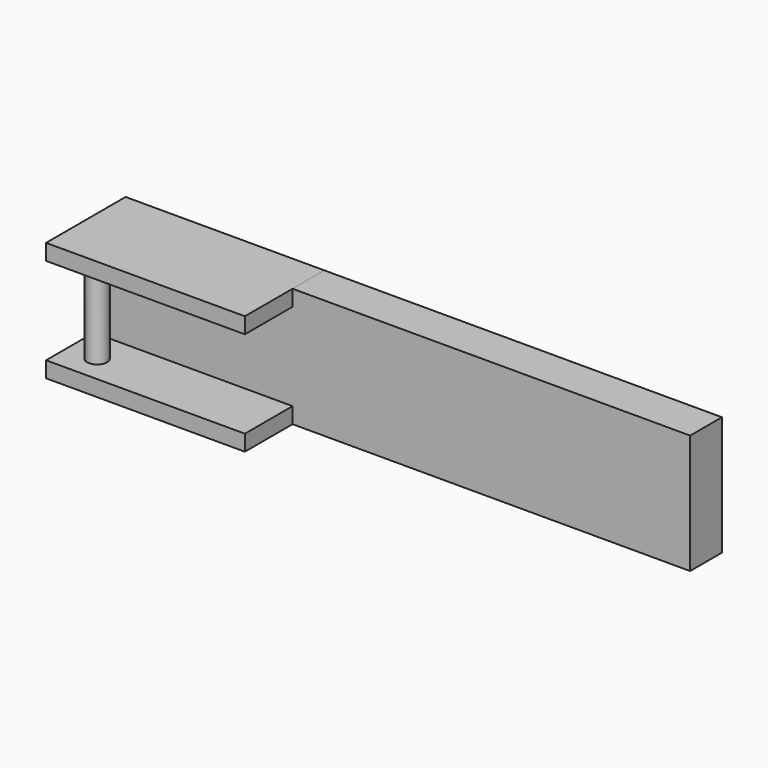
from build123d import *

# Parameters (mm, degrees)
F0_W     = 63.5
F0_H     = 5.08
F1_DEPTH = 31.75
F0_H_2   = 27.94
F2_DEPTH = 12.7
F3_R     = 3.175
F4_DEPTH = 28.702


with BuildPart() as f1:
    # F0 (on Front) → F1 (new body)
    with BuildSketch(Plane.XZ):
        with Locations((-63.5, 16.51)):
            Rectangle(F0_W, F0_H)
    extrude(amount=F1_DEPTH)

    # F3 (on face) → F4 (join)
    with BuildSketch(Plane(origin=(0, 0, 13.97), x_dir=(1, 0, 0), z_dir=(0, 0, -1))):
        with Locations((-85.8540832996, 23.1188889593)):
            Circle(F3_R)
    extrude(amount=F4_DEPTH)


with BuildPart() as f1b:
    # F0 (on Front) → F1, piece 2 (new body)
    with BuildSketch(Plane.XZ):
        with Locations((-63.5, -16.51)):
            Rectangle(F0_W, F0_H)
    extrude(amount=F1_DEPTH)


with BuildPart() as f2:
    # F0 (on Front) → F2 (new body)
    with BuildSketch(Plane.XZ):
        with Locations((-63.5, 0)):
            Rectangle(F0_W, F0_H_2)
        Polygon((95.25, -19.05), (95.25, 19.05), (-31.75, 19.05), (-31.75, 13.97), (-31.75, -13.97), (-31.75, -19.05), align=None)
    extrude(amount=F2_DEPTH)


solid = Compound([f1.part, f1b.part, f2.part])
